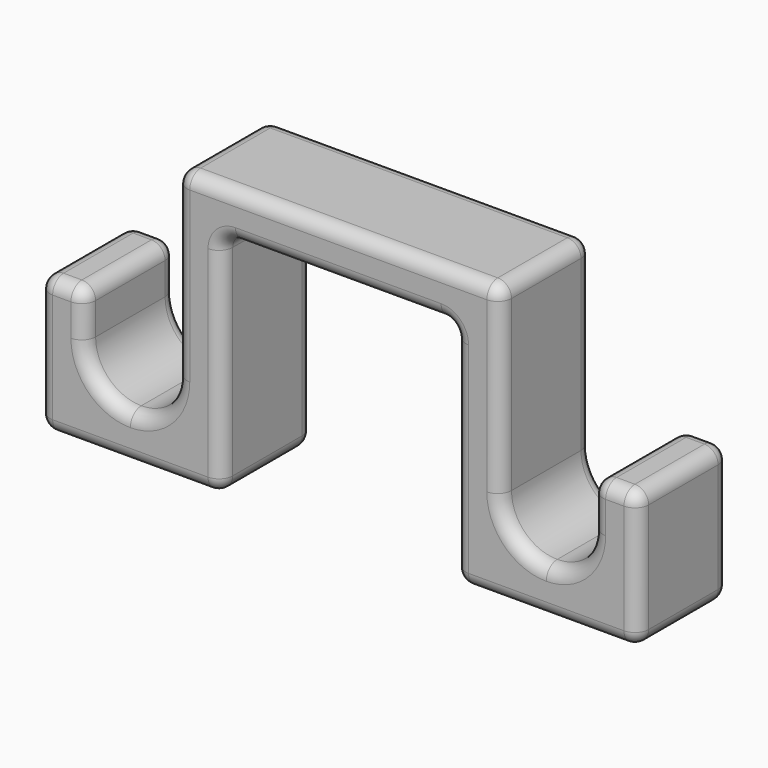
from build123d import *

# Parameters (mm, degrees)
F1_DEPTH = 25
F2_R     = 3
F3_R     = 9.99999
F5_R     = 3


# Not quite as in the source:
# - a fillet or chamfer is up to 0.001 mm smaller than in the source, because OpenCascade refuses the exact size


with BuildPart() as f1:
    # F0 (on Front) → F1 (new body)
    with BuildSketch(Plane.XZ):
        Polygon((-10, 0), (0, 0), (0, 60), (-71, 60), (-71, 10), (-91, 10), (-91, 30), (-101, 30), (-101, 0), (-61, 0), (-61, 50), (-10, 50), align=None)
    extrude(amount=F1_DEPTH)

    # F2
    f2_edges = [f1.edges().sort_by_distance(p)[0] for p in [
        (-71, -12.5, 60),
        (0, -12.5, 60),
        (-10, -12.5, 50),
        (-61, -12.5, 50),
        (-61, -12.5, 0),
        (-10, -12.5, 0),
        (0, -12.5, 0),
        (-101, -12.5, 0),
        (-101, -12.5, 30),
        (-91, -12.5, 30),
    ]]
    fillet(f2_edges, radius=F2_R)

    # F3 (radius 10 in the source; OpenCascade refuses exactly that, so slightly less here)
    f3_edges = [f1.edges().sort_by_distance(p)[0] for p in [
        (-91, -12.5, 10),
        (-71, -12.5, 10),
    ]]
    fillet(f3_edges, radius=F3_R)

    # F5
    f5_edges = [f1.edges().sort_by_distance(p)[0] for p in [
        (-71, -25, 38.499995),
        (-73.928929, -25, 12.928929),
        (-70.12132, -25, 59.12132),
        (-81, -25, 10),
        (-35.5, -25, 60),
        (-88.071071, -25, 12.928929),
        (-0.87868, -25, 59.12132),
        (-91, -25, 23.499995),
        (0, -25, 30),
        (-91.87868, -25, 29.12132),
        (-0.87868, -25, 0.87868),
        (-96, -25, 30),
        (-5, -25, 0),
        (-100.12132, -25, 29.12132),
        (-9.12132, -25, 0.87868),
        (-101, -25, 15),
        (-10, -25, 25),
        (-100.12132, -25, 0.87868),
        (-10.87868, -25, 49.12132),
        (-81, -25, 0),
        (-35.5, -25, 50),
        (-61.87868, -25, 0.87868),
        (-60.12132, -25, 49.12132),
        (-61, -25, 25),
        (-71, 0, 38.499995),
        (-73.928929, 0, 12.928929),
        (-70.12132, 0, 59.12132),
        (-81, 0, 10),
        (-35.5, 0, 60),
        (-88.071071, 0, 12.928929),
        (-0.87868, 0, 59.12132),
        (-91, 0, 23.499995),
        (0, 0, 30),
        (-91.87868, 0, 29.12132),
        (-0.87868, 0, 0.87868),
        (-96, 0, 30),
        (-5, 0, 0),
        (-100.12132, 0, 29.12132),
        (-9.12132, 0, 0.87868),
        (-101, 0, 15),
        (-10, 0, 25),
        (-100.12132, 0, 0.87868),
        (-10.87868, 0, 49.12132),
        (-81, 0, 0),
        (-35.5, 0, 50),
        (-61.87868, 0, 0.87868),
        (-60.12132, 0, 49.12132),
        (-61, 0, 25),
    ]]
    fillet(f5_edges, radius=F5_R)

    # F6: F1 across plane


with BuildPart() as f1_1:
    add(f1.part)
    add(f1.part.mirror(Plane(origin=(-35.5, -12.5, 34.2499975), x_dir=(0, 1, 0), z_dir=(1, 0, 0))))


solid = f1_1.part
